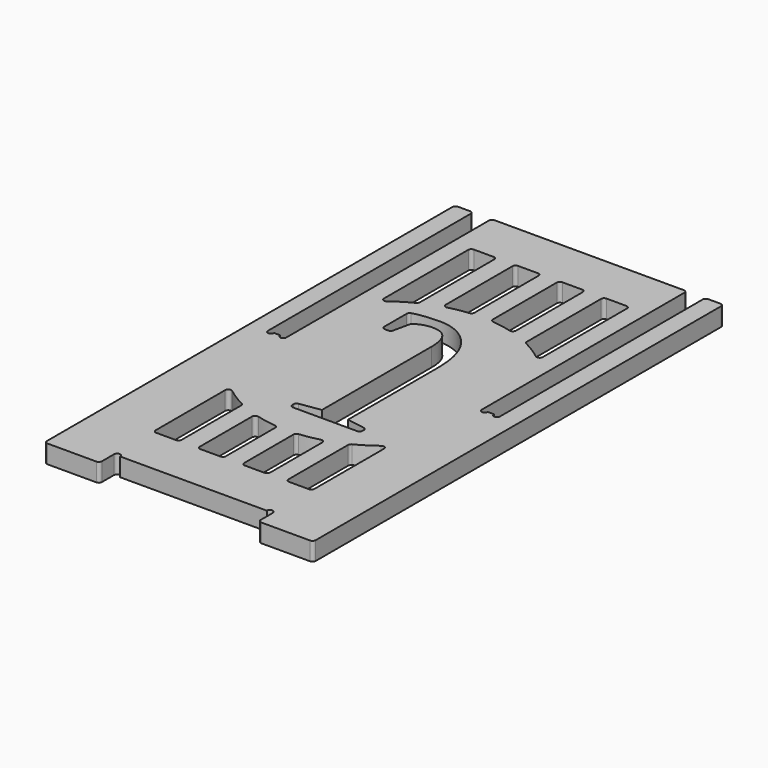
from build123d import *

# Parameters (mm, degrees)
F2_DEPTH     = 19.05
F3_R         = 3.175
F5_DEPTH     = 19.05
F6_TEXT_SIZE = 289.9994866716
F7_DEPTH     = 25.4
F8_R         = 3.175


# Not quite as in the source:
# - Text() gives the source's letters only with a copy of the font that has no kerning and outlines rounded to 1/6400 em; it was checked with that copy


with BuildPart() as f2:
    # F1 (on offset) → F2 (new body)
    with BuildSketch(Plane.XY.offset(19.05)):
        Polygon((0, 514.35), (0, -19.05), (57.15, -19.05), (57.15, 0), (222.25, 0), (222.25, -19.05), (279.4, -19.05), (279.4, 514.35), (260.35, 514.35), (260.35, 247.65), (241.3, 247.65), (241.3, 514.35), (38.1, 514.35), (38.1, 247.65), (19.05, 247.65), (19.05, 514.35), align=None)
    extrude(amount=F2_DEPTH)

    # F3
    f3_edges = [f2.edges().sort_by_distance(p)[0] for p in [
        (0, -19.05, 28.575),
        (57.15, -19.05, 28.575),
        (222.25, -19.05, 28.575),
        (279.4, -19.05, 28.575),
        (0, 514.35, 28.575),
        (19.05, 514.35, 28.575),
        (38.1, 514.35, 28.575),
        (241.3, 514.35, 28.575),
        (260.35, 514.35, 28.575),
        (279.4, 514.35, 28.575),
    ]]
    fillet(f3_edges, radius=F3_R)

    # F4 (on face) → F5 (cut)
    with BuildSketch(Plane(origin=(0, 0, 19.05), x_dir=(1, 0, 0), z_dir=(0, 0, -1))):
        with BuildLine():
            Line((63.5, 0), (57.15, 0))
            ThreePointArc((57.15, 0), (60.325, -3.175), (63.5, 0))
        make_face()
        with BuildLine():
            ThreePointArc((215.9, 0), (219.075, -3.175), (222.25, 0))
            Line((222.25, 0), (215.9, 0))
        make_face()
        with BuildLine():
            ThreePointArc((25.4, -247.65), (22.225, -244.475), (19.05, -247.65))
            Line((19.05, -247.65), (25.4, -247.65))
        make_face()
        with BuildLine():
            Line((31.75, -247.65), (38.1, -247.65))
            ThreePointArc((38.1, -247.65), (34.925, -244.475), (31.75, -247.65))
        make_face()
        with BuildLine():
            ThreePointArc((247.65, -247.65), (244.475, -244.475), (241.3, -247.65))
            Line((241.3, -247.65), (247.65, -247.65))
        make_face()
        with BuildLine():
            Line((254, -247.65), (260.35, -247.65))
            ThreePointArc((260.35, -247.65), (257.175, -244.475), (254, -247.65))
        make_face()
    extrude(amount=-F5_DEPTH, mode=Mode.SUBTRACT)

    # F6 (on face) → F7 (cut)
    with BuildSketch(Plane(origin=(0, 0, 19.05), x_dir=(1, 0, 0), z_dir=(0, 0, -1))):
        with BuildLine():
            Line((57.15, -50.8), (57.15, -151.1383556248))
            ThreePointArc((57.15, -151.1383556248), (70.0796604885, -141.4332012989), (84.1375, -133.4492618511))
            Line((84.1375, -133.4492618511), (84.1375, -50.8))
            Line((84.1375, -50.8), (57.15, -50.8))
        make_face()
        with BuildLine():
            Line((103.1875, -50.8), (103.1875, -126.011859009))
            ThreePointArc((103.1875, -126.011859009), (116.5456640044, -122.7785592115), (130.175, -121.0076912126))
            Line((130.175, -121.0076912126), (130.175, -50.8))
            Line((130.175, -50.8), (103.1875, -50.8))
        make_face()
        with BuildLine():
            Line((149.225, -50.8), (149.225, -121.0076912126))
            ThreePointArc((149.225, -121.0076912126), (162.8543359956, -122.7785592115), (176.2125, -126.011859009))
            Line((176.2125, -126.011859009), (176.2125, -50.8))
            Line((176.2125, -50.8), (149.225, -50.8))
        make_face()
        with BuildLine():
            Line((195.2625, -50.8), (195.2625, -133.4492618511))
            ThreePointArc((195.2625, -133.4492618511), (209.3203395115, -141.4332012989), (222.25, -151.1383556248))
            Line((222.25, -151.1383556248), (222.25, -50.8))
            Line((222.25, -50.8), (195.2625, -50.8))
        make_face()
        with BuildLine():
            ThreePointArc((84.1375, -361.8507381489), (70.0796604885, -353.8667987011), (57.15, -344.1616443752))
            Line((57.15, -344.1616443752), (57.15, -463.55))
            Line((57.15, -463.55), (84.1375, -463.55))
            Line((84.1375, -463.55), (84.1375, -361.8507381489))
        make_face()
        with BuildLine():
            ThreePointArc((130.175, -374.2923087874), (116.5456640044, -372.5214407885), (103.1875, -369.288140991))
            Line((103.1875, -369.288140991), (103.1875, -463.55))
            Line((103.1875, -463.55), (130.175, -463.55))
            Line((130.175, -463.55), (130.175, -374.2923087874))
        make_face()
        with BuildLine():
            Line((149.225, -374.2923087874), (149.225, -463.55))
            Line((149.225, -463.55), (176.2125, -463.55))
            Line((176.2125, -463.55), (176.2125, -369.288140991))
            ThreePointArc((176.2125, -369.288140991), (162.8543359956, -372.5214407885), (149.225, -374.2923087874))
        make_face()
        with BuildLine():
            ThreePointArc((222.25, -344.1616443752), (209.3203395115, -353.8667987011), (195.2625, -361.8507381489))
            Line((195.2625, -361.8507381489), (195.2625, -463.55))
            Line((195.2625, -463.55), (222.25, -463.55))
            Line((222.25, -463.55), (222.25, -344.1616443752))
        make_face()
        with Locations((82.2265595198, -344.9275046587)):
            Text('J', F6_TEXT_SIZE, font='Tinos', text_align=(TextAlign.LEFT, TextAlign.BOTTOM))
    extrude(amount=-F7_DEPTH, mode=Mode.SUBTRACT)

    # F8
    f8_edges = [f2.edges().sort_by_distance(p)[0] for p in [
        (57.15, 50.8, 28.575),
        (103.1875, 50.8, 28.575),
        (149.225, 50.8, 28.575),
        (195.2625, 50.8, 28.575),
        (84.1375, 50.8, 28.575),
        (130.175, 50.8, 28.575),
        (176.2125, 50.8, 28.575),
        (222.25, 50.8, 28.575),
        (57.15, 151.138356, 28.575),
        (103.1875, 126.011859, 28.575),
        (149.225, 121.007691, 28.575),
        (195.2625, 133.449262, 28.575),
        (84.1375, 133.449262, 28.575),
        (130.175, 121.007691, 28.575),
        (176.2125, 126.011859, 28.575),
        (222.25, 151.138356, 28.575),
        (84.1375, 463.55, 28.575),
        (130.175, 463.55, 28.575),
        (176.2125, 463.55, 28.575),
        (222.25, 463.55, 28.575),
        (195.2625, 463.55, 28.575),
        (149.225, 463.55, 28.575),
        (103.1875, 463.55, 28.575),
        (57.15, 463.55, 28.575),
        (84.1375, 361.850738, 28.575),
        (130.175, 374.292309, 28.575),
        (176.2125, 369.288141, 28.575),
        (222.25, 344.161644, 28.575),
        (195.2625, 361.850738, 28.575),
        (149.225, 374.292309, 28.575),
        (103.1875, 369.288141, 28.575),
        (57.15, 344.161644, 28.575),
        (88.298424, 308.949443, 28.575),
        (97.678095, 308.949443, 28.575),
        (88.298424, 343.52282, 28.575),
        (188.982621, 155.023153, 28.575),
        (188.982621, 162.545015, 28.575),
        (115.939, 155.023153, 28.575),
        (115.939, 162.545015, 28.575),
    ]]
    fillet(f8_edges, radius=F8_R)


solid = f2.part
